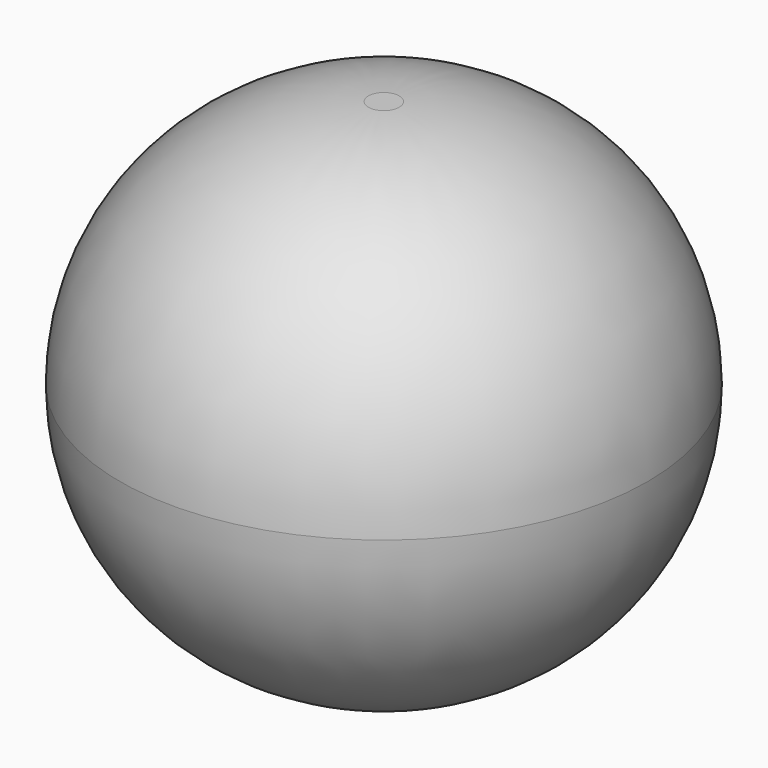
from build123d import *

# Parameters (mm, degrees)
F0_R     = 53.9454958118
F1_DEPTH = 101.6
F2_R     = 50.79999


# Not quite as in the source:
# - a fillet or chamfer is up to 0.001 mm smaller than in the source, because OpenCascade refuses the exact size


with BuildPart() as f1:
    # F0 (on Top) → F1 (new body)
    with BuildSketch(Plane.XY):
        with Locations((-0.1693964005, -0.1693889499)):
            Circle(F0_R)
    extrude(amount=F1_DEPTH)

    # F2 (radius 50.8 in the source; OpenCascade refuses exactly that, so slightly less here)
    f2_edges = [f1.edges().sort_by_distance(p)[0] for p in [
        (-54.114892, -0.169389, 101.6),
        (-54.114892, -0.169389, 0),
    ]]
    fillet(f2_edges, radius=F2_R)


solid = f1.part
